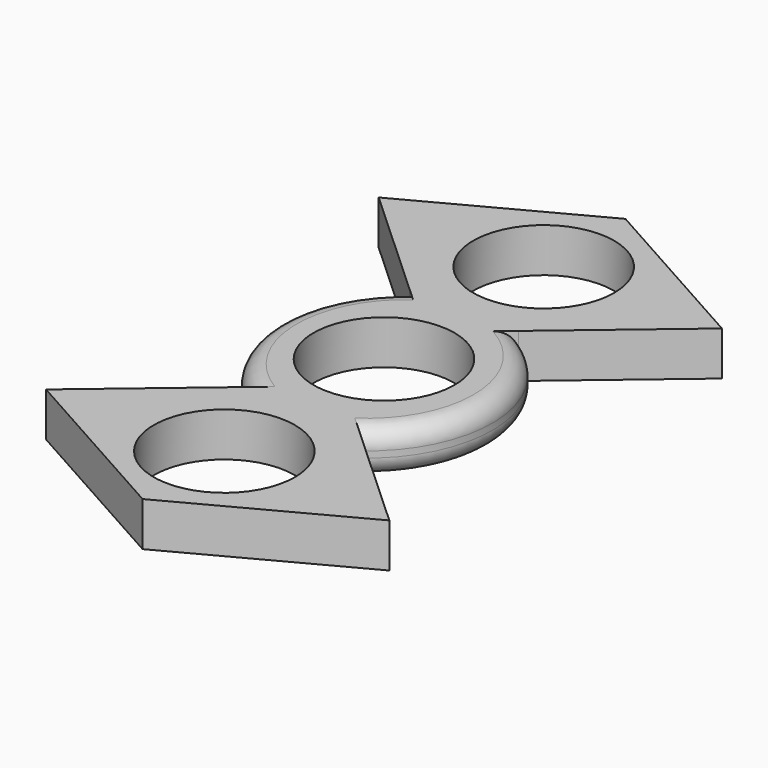
from build123d import *

# Parameters (mm, degrees)
F0_R         = 11.2
F1_DEPTH     = 7
F2_T4_ANGLE  = 151.1667099625
F2_T10_ANGLE = 155.7575231718
F2_T16_ANGLE = 151.1667099625
F2_T22_ANGLE = 155.7575231718


# Not quite as in the source:
# - a fillet or chamfer that OpenCascade refuses, or shapes differently, is made with other operations: its cross-section is extruded or revolved along the edge and cut away or added


with BuildPart() as f1:
    # F0 (on Top) → F1 (new body)
    with BuildSketch(Plane.XY):
        with BuildLine():
            ThreePointArc((9.3591465956, -16.7270162039), (17.6571466732, 0.0595617509), (8.3139799998, 16.2876621091))
            Line((8.3139799998, 16.2876621091), (-9.3591465956, 16.7270162039))
            ThreePointArc((-9.3591465956, 16.7270162039), (-17.3223324531, -0.048962325), (-8.3139799998, -16.2876621091))
            Line((-8.3139799998, -16.2876621091), (9.3591465956, -16.7270162039))
        make_face()
        Circle(F0_R, mode=Mode.SUBTRACT)
        Polygon((8.3139799998, 16.2876621091), (27.5946892798, 32.5588136911), (-0.1261595724, 48.0615143736), (-27.5946892798, 33.4348380566), (-9.3591465956, 16.7270162039), align=None)
        with Locations((0, 31.6827967763)):
            Circle(F0_R, mode=Mode.SUBTRACT)
        Polygon((27.5946892798, -33.4348380566), (9.3591465956, -16.7270162039), (-8.3139799998, -16.2876621091), (-27.5946892798, -32.5588136911), (0.1261595724, -48.0615143736), align=None)
        with Locations((0, -31.6827967763)):
            Circle(F0_R, mode=Mode.SUBTRACT)
    extrude(amount=F1_DEPTH)

    # F2: fillet of radius 3 on 4 edges, made by hand


with BuildPart() as f2_tool2:
    # F2_s3 → F2_t4 (revolve)
    with BuildSketch(Plane(origin=(2.9031932082, 0.8450981198, 0), x_dir=(0, 0, 1), z_dir=(0.9601480198, 0.2794920035, 0))):
        with BuildLine():
            ThreePointArc((4, -20.0470026749), (6.1213203436, -19.1683230184), (7, -17.0470026749))
            Line((7, -17.0470026749), (7, -20.0470026749))
            Line((7, -20.0470026749), (4, -20.0470026749))
        make_face()
    revolve(axis=Axis((2.9763887281, 0.5936471566, 7), (0, 0, 1)), revolution_arc=F2_T4_ANGLE)

    split(bisect_by=Plane(origin=(4.0604237069, 4.4316985467, 0), x_dir=(0, 0, 1), z_dir=(-0.6755468125, -0.7373170987, 0)), keep=Keep.TOP)

    split(bisect_by=Plane(origin=(4.569745577, -5.414978498, 0), x_dir=(0, 0, 1), z_dir=(-0.6449416276, 0.7642318346, 0)), keep=Keep.TOP)


with BuildPart() as f1_1:
    add(f1.part)

    # F2_t1: cut F2_tool2
    add(f2_tool2.part, mode=Mode.SUBTRACT)


with BuildPart() as f2_tool8:
    # F2_s9 → F2_t10 (revolve)
    with BuildSketch(Plane(origin=(-2.2049800931, -0.547085883, 0), x_dir=(0, 0, 1), z_dir=(-0.9705717322, -0.2408121936, 0))):
        with BuildLine():
            ThreePointArc((4, -19.889257837), (6.1213203436, -19.0105781805), (7, -16.889257837))
            Line((7, -16.889257837), (7, -19.889257837))
            Line((7, -19.889257837), (4, -19.889257837))
        make_face()
    revolve(axis=Axis((-2.1995295918, -0.5690536346, 7), (0, 0, 1)), revolution_arc=F2_T10_ANGLE)

    split(bisect_by=Plane(origin=(-4.0604237069, -4.4316985467, 0), x_dir=(0, 0, 1), z_dir=(0.6755468125, 0.7373170987, 0)), keep=Keep.TOP)

    split(bisect_by=Plane(origin=(-4.569745577, 5.414978498, 0), x_dir=(0, 0, 1), z_dir=(0.6449416276, -0.7642318346, 0)), keep=Keep.TOP)


with BuildPart() as f1_2:
    add(f1_1.part)

    # F2_t7: cut F2_tool8
    add(f2_tool8.part, mode=Mode.SUBTRACT)


with BuildPart() as f2_tool14:
    # F2_s15 → F2_t16 (revolve)
    with BuildSketch(Plane(origin=(2.9031932082, 0.8450981198, 0), x_dir=(0, 0, 1), z_dir=(0.9601480198, 0.2794920035, 0))):
        with BuildLine():
            ThreePointArc((3, -20.0470026749), (0.8786796564, -19.1683230184), (0, -17.0470026749))
            Line((0, -17.0470026749), (0, -20.0470026749))
            Line((0, -20.0470026749), (3, -20.0470026749))
        make_face()
    revolve(axis=Axis((2.9763887281, 0.5936471566, 0), (0, 0, 1)), revolution_arc=F2_T16_ANGLE)

    split(bisect_by=Plane(origin=(4.0604237069, 4.4316985467, 0), x_dir=(0, 0, 1), z_dir=(-0.6755468125, -0.7373170987, 0)), keep=Keep.TOP)

    split(bisect_by=Plane(origin=(4.569745577, -5.414978498, 0), x_dir=(0, 0, 1), z_dir=(-0.6449416276, 0.7642318346, 0)), keep=Keep.TOP)


with BuildPart() as f1_3:
    add(f1_2.part)

    # F2_t13: cut F2_tool14
    add(f2_tool14.part, mode=Mode.SUBTRACT)


with BuildPart() as f2_tool20:
    # F2_s21 → F2_t22 (revolve)
    with BuildSketch(Plane(origin=(-2.2049800931, -0.547085883, 0), x_dir=(0, 0, 1), z_dir=(-0.9705717322, -0.2408121936, 0))):
        with BuildLine():
            ThreePointArc((3, -19.889257837), (0.8786796564, -19.0105781805), (0, -16.889257837))
            Line((0, -16.889257837), (0, -19.889257837))
            Line((0, -19.889257837), (3, -19.889257837))
        make_face()
    revolve(axis=Axis((-2.1995295918, -0.5690536346, 0), (0, 0, 1)), revolution_arc=F2_T22_ANGLE)

    split(bisect_by=Plane(origin=(-4.0604237069, -4.4316985467, 0), x_dir=(0, 0, 1), z_dir=(0.6755468125, 0.7373170987, 0)), keep=Keep.TOP)

    split(bisect_by=Plane(origin=(-4.569745577, 5.414978498, 0), x_dir=(0, 0, 1), z_dir=(0.6449416276, -0.7642318346, 0)), keep=Keep.TOP)


with BuildPart() as f1_4:
    add(f1_3.part)

    # F2_t19: cut F2_tool20
    add(f2_tool20.part, mode=Mode.SUBTRACT)


solid = f1_4.part
